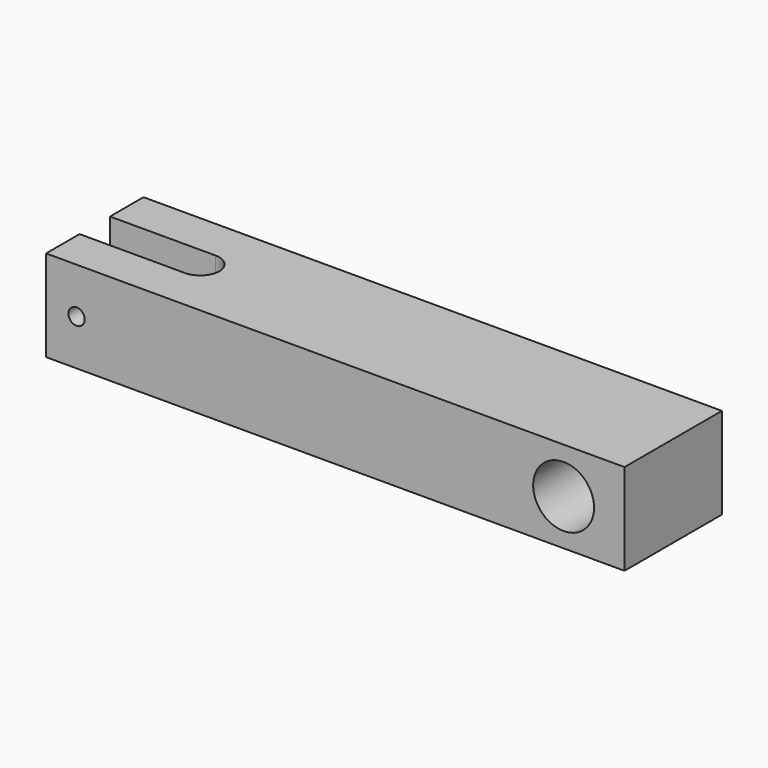
from build123d import *

# Parameters (mm, degrees)
F0_W     = 60.325
F0_H     = 9.525
F0_R     = 0.8509
F0_R_2   = 3.175
F1_DEPTH = 12.7
F3_DEPTH = 9.526


# Not quite as in the source:
# - a feature of the source that left no trace in its solid (it failed there, or was rolled back) is left out


with BuildPart() as f1:
    # F0 (on Front) → F1 (new body)
    with BuildSketch(Plane.XZ):
        with Locations((30.1625, 4.7625)):
            Rectangle(F0_W, F0_H)
        with Locations((3.175, 4.7625)):
            Circle(F0_R, mode=Mode.SUBTRACT)
        with Locations((53.975, 4.7625)):
            Circle(F0_R_2, mode=Mode.SUBTRACT)
    extrude(amount=-F1_DEPTH)

    # F2 (on face) → F3 (cut, through all)
    with BuildSketch(Plane.XY.offset(9.525)):
        with BuildLine():
            Line((10.99566, 8.33374), (0, 8.33374))
            Line((0, 8.33374), (0, 4.36626))
            Line((0, 4.36626), (10.99566, 4.36626))
            ThreePointArc((10.99566, 4.36626), (12.3983760061, 4.9472839939), (12.9794, 6.35))
            ThreePointArc((12.9794, 6.35), (12.3983760061, 7.7527160061), (10.99566, 8.33374))
        make_face()
    extrude(amount=-F3_DEPTH, mode=Mode.SUBTRACT)


solid = f1.part
